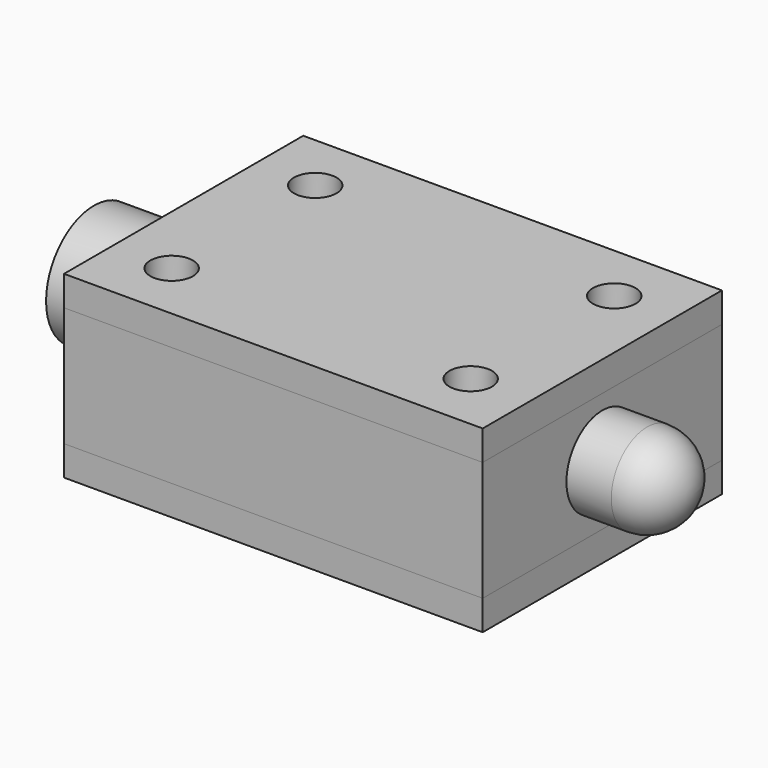
from build123d import *

# Parameters (mm, degrees)
F0_W            = 22.225
F0_H            = 15.875
F1_DEPTH        = 6.35
F3_D            = 2.2606
F4_R            = 3.175
F5_DEPTH        = 4.7625
F7_R            = 2.38125
F8_DEPTH        = 4.7625
F9_R            = 2.38125
F12_D           = 1.5875
F12_DEPTH       = 7.14375
F12_TIP         = 0.4769331164
F14_D           = 2.4384
F14_DEPTH       = 11.1125
F14_CBORE_D     = 4.0386
F14_CBORE_DEPTH = 6.35
F14_TIP         = 0.7325692667
F15_R           = 1.524
F16_DEPTH       = 3.571875
F18_W           = 22.225
F18_H           = 15.875
F18_R           = 1.1303
F18_R_2         = 0.5461
F19_DEPTH       = 1.5875
F21_W           = 22.225
F21_H           = 15.875
F21_R           = 1.1303
F22_DEPTH       = 1.5875


with BuildPart() as f1:
    # F0 (on Top) → F1 (new body)
    with BuildSketch(Plane.XY):
        Rectangle(F0_W, F0_H)
        with BuildLine():
            ThreePointArc((-6.746875, 2.181225), (-6.1070790528, 3.7258290528), (-4.562475, 4.365625))
            Line((-4.562475, 4.365625), (4.562475, 4.365625))
            ThreePointArc((4.562475, 4.365625), (6.1070790528, 3.7258290528), (6.746875, 2.181225))
            Line((6.746875, 2.181225), (6.746875, -2.181225))
            ThreePointArc((6.746875, -2.181225), (6.1070790528, -3.7258290528), (4.562475, -4.365625))
            Line((4.562475, -4.365625), (-4.562475, -4.365625))
            ThreePointArc((-4.562475, -4.365625), (-6.1070790528, -3.7258290528), (-6.746875, -2.181225))
            Line((-6.746875, -2.181225), (-6.746875, 2.181225))
        make_face(mode=Mode.SUBTRACT)
    extrude(amount=F1_DEPTH)

    # F3 (through all)
    with Locations(Plane.XY.offset(6.35)):
        with Locations((-7.9375, 4.7625), (7.9375, 4.7625), (7.9375, -4.7625), (-7.9375, -4.7625)):
            Hole(F3_D / 2)

    # F4 (on face) → F5 (join)
    with BuildSketch(Plane(origin=(-11.1125, 0, 0), x_dir=(0, -1, 0), z_dir=(-1, 0, 0))):
        with Locations((0, 3.175)):
            Circle(F4_R)
    extrude(amount=F5_DEPTH)

    # F7 (on face) → F8 (join)
    with BuildSketch(Plane.YZ.offset(11.1125)):
        with Locations((0, 3.175)):
            Circle(F7_R)
    extrude(amount=F8_DEPTH)

    # F9
    f9_edges = [f1.edges().sort_by_distance(p)[0] for p in [
        (15.875, -2.38125, 3.175),
    ]]
    fillet(f9_edges, radius=F9_R)

    # F12 (one way)
    with BuildSketch(Plane(origin=(6.746875, 0, 0), x_dir=(0, -1, 0), z_dir=(-1, 0, 0))):
        with Locations((0, 3.175)):
            Circle(F12_D / 2)
    extrude(amount=-F12_DEPTH, mode=Mode.SUBTRACT)
    with Locations(Plane(origin=(6.746875, 0, 0), x_dir=(0, -1, 0), z_dir=(-1, 0, 0))):
        with Locations((0, 3.175)):
            with Locations((0, 0, -(F12_DEPTH + F12_TIP / 2))):  # 118° drill point
                Cone(0, F12_D / 2, F12_TIP, mode=Mode.SUBTRACT)

    # F14
    with Locations(Plane(origin=(-15.875, 0, 0), x_dir=(0, -1, 0), z_dir=(-1, 0, 0))):
        with Locations((0, 3.175)):
            CounterBoreHole(F14_D / 2, F14_CBORE_D / 2, F14_CBORE_DEPTH, depth=F14_DEPTH)
            with Locations((0, 0, -(F14_DEPTH + F14_TIP / 2))):  # 118° drill point
                Cone(0, F14_D / 2, F14_TIP, mode=Mode.SUBTRACT)

    # F15 (on face) → F16 (cut, through all)
    with BuildSketch(Plane(origin=(0, 7.9375, 0), x_dir=(-1, 0, 0), z_dir=(0, 1, 0))):
        with Locations((0, 3.175)):
            Circle(F15_R)
    extrude(amount=-F16_DEPTH, mode=Mode.SUBTRACT)


with BuildPart() as f1_1:
    # F17: moved
    add(f1.part.moved(Location((0, 0, 1.5875))))


with BuildPart() as f19:
    # F18 (on Top) → F19 (new body)
    with BuildSketch(Plane.XY):
        Rectangle(F18_W, F18_H)
        with Locations((-7.9375, -4.7625)):
            Circle(F18_R, mode=Mode.SUBTRACT)
        with Locations((-2.54, -1.5875)):
            Circle(F18_R_2, mode=Mode.SUBTRACT)
        with Locations((7.9375, -4.7625)):
            Circle(F18_R, mode=Mode.SUBTRACT)
        with Locations((0, -1.5875)):
            Circle(F18_R_2, mode=Mode.SUBTRACT)
        with Locations((2.54, -1.5875)):
            Circle(F18_R_2, mode=Mode.SUBTRACT)
        with Locations((-2.54, 0)):
            Circle(F18_R_2, mode=Mode.SUBTRACT)
        with Locations((-2.54, 1.5875)):
            Circle(F18_R_2, mode=Mode.SUBTRACT)
        with Locations((-7.9375, 4.7625)):
            Circle(F18_R, mode=Mode.SUBTRACT)
        Circle(F18_R_2, mode=Mode.SUBTRACT)
        with Locations((2.54, 0)):
            Circle(F18_R_2, mode=Mode.SUBTRACT)
        with Locations((0, 1.5875)):
            Circle(F18_R_2, mode=Mode.SUBTRACT)
        with Locations((2.54, 1.5875)):
            Circle(F18_R_2, mode=Mode.SUBTRACT)
        with Locations((7.9375, 4.7625)):
            Circle(F18_R, mode=Mode.SUBTRACT)
    extrude(amount=F19_DEPTH)


with BuildPart() as f22:
    # F21 (on offset) → F22 (new body)
    with BuildSketch(Plane.XY.offset(7.9375)):
        Rectangle(F21_W, F21_H)
        with Locations((-7.9375, -4.7625)):
            Circle(F21_R, mode=Mode.SUBTRACT)
        with Locations((7.9375, -4.7625)):
            Circle(F21_R, mode=Mode.SUBTRACT)
        with Locations((-7.9375, 4.7625)):
            Circle(F21_R, mode=Mode.SUBTRACT)
        with Locations((7.9375, 4.7625)):
            Circle(F21_R, mode=Mode.SUBTRACT)
    extrude(amount=F22_DEPTH)


solid = Compound([f1_1.part, f19.part, f22.part])
